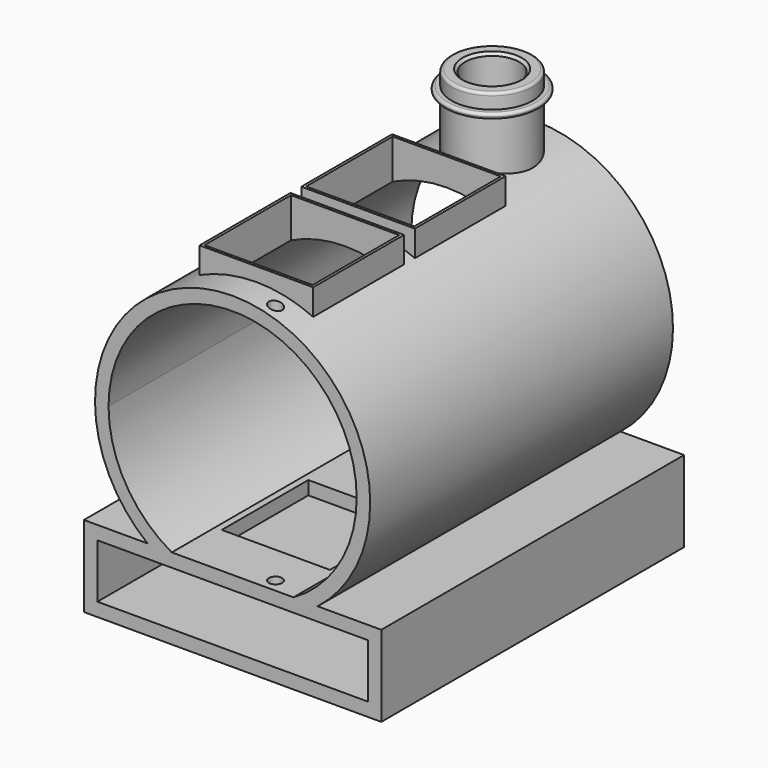
from build123d import *

# Parameters (mm, degrees)
F0_W      = 5
F0_H      = 5
F1_DEPTH  = 140
F5_R      = 15
F5_R_2    = 10
F6_DEPTH  = 30
F7_R      = 10
F8_DEPTH  = 25
F7_W      = 42
F7_H      = 42
F7_W_2    = 40
F7_H_2    = 40
F9_DEPTH  = 10
F10_DEPTH = 25
F11_W     = 40
F11_H     = 40
F11_R     = 2.4384
F11_R_2   = 2.4765
F12_DEPTH = 25
F13_DEPTH = 100
F15_R     = 17.5
F15_R_2   = 10
F16_DEPTH = 2
F17_R     = 0.99999
F18_SIZE  = 1


# Not quite as in the source:
# - a fillet or chamfer is up to 0.001 mm smaller than in the source, because OpenCascade refuses the exact size


with BuildPart() as f1:
    # F0 (on Front) → F1 (new body)
    with BuildSketch(Plane.XZ):
        with BuildLine():
            ThreePointArc((-22.5, -40), (-39.6160493738, -23.1693468188), (-45.8938993767, 0))
            Line((-45.8938993767, 0), (-50.8938993767, 0))
            ThreePointArc((-50.8938993767, 0), (-45.7803505669, -22.233949171), (-31.4672686099, -40))
            Line((-31.4672686099, -40), (-22.5, -40))
        make_face()
        with BuildLine():
            ThreePointArc((-9.0138781887, -45), (-15.954031767, -43.0316031583), (-22.5, -40))
            Line((-22.5, -40), (-31.4672686099, -40))
            ThreePointArc((-31.4672686099, -40), (-27.7333960958, -42.6737358894), (-23.7737038294, -45))
            Line((-23.7737038294, -45), (-9.0138781887, -45))
        make_face()
        with BuildLine():
            ThreePointArc((-45.8938993767, 0), (0, 45.8938993767), (45.8938993767, 0))
            Line((45.8938993767, 0), (50.8938993767, 0))
            ThreePointArc((50.8938993767, 0), (0, 50.8938993767), (-50.8938993767, 0))
            Line((-50.8938993767, 0), (-45.8938993767, 0))
        make_face()
        with BuildLine():
            Line((50.8938993767, 0), (45.8938993767, 0))
            ThreePointArc((45.8938993767, 0), (39.6160493738, -23.1693468188), (22.5, -40))
            Line((22.5, -40), (31.4672686099, -40))
            ThreePointArc((31.4672686099, -40), (45.7803505669, -22.233949171), (50.8938993767, 0))
        make_face()
        with Locations((-52.5, -67.5)):
            Rectangle(F0_W, F0_H)
        with BuildLine():
            ThreePointArc((-23.7737038294, -45), (-27.7333960958, -42.6737358894), (-31.4672686099, -40))
            Line((-31.4672686099, -40), (-55, -40))
            Line((-55, -40), (-55, -65))
            Line((-55, -65), (-50, -65))
            Line((-50, -65), (-50, -45))
            Line((-50, -45), (-23.7737038294, -45))
        make_face()
        with BuildLine():
            Line((55, -40), (31.4672686099, -40))
            ThreePointArc((31.4672686099, -40), (27.7333960958, -42.6737358894), (23.7737038294, -45))
            Line((23.7737038294, -45), (50, -45))
            Line((50, -45), (50, -65))
            Line((50, -65), (-50, -65))
            Line((-50, -65), (-50, -70))
            Line((-50, -70), (55, -70))
            Line((55, -70), (55, -40))
        make_face()
        with BuildLine():
            ThreePointArc((9.0138781887, -45), (15.954031767, -43.0316031583), (22.5, -40))
            Line((22.5, -40), (0, -40))
            Line((0, -40), (-22.5, -40))
            ThreePointArc((-22.5, -40), (-15.954031767, -43.0316031583), (-9.0138781887, -45))
            Line((-9.0138781887, -45), (9.0138781887, -45))
        make_face()
        with BuildLine():
            Line((31.4672686099, -40), (22.5, -40))
            ThreePointArc((22.5, -40), (15.954031767, -43.0316031583), (9.0138781887, -45))
            Line((9.0138781887, -45), (23.7737038294, -45))
            ThreePointArc((23.7737038294, -45), (27.7333960958, -42.6737358894), (31.4672686099, -40))
        make_face()
    extrude(amount=F1_DEPTH)

    # F5 (on offset) → F6 (join)
    with BuildSketch(Plane.XY.offset(76)):
        with Locations((0, -20)):
            Circle(F5_R)
        with Locations((0, -20)):
            Circle(F5_R_2, mode=Mode.SUBTRACT)
    extrude(amount=-F6_DEPTH)

    # F7 (on offset) → F8 (cut)
    with BuildSketch(Plane.XY.offset(56)):
        with Locations((0, -20)):
            Circle(F7_R)
    extrude(amount=-F8_DEPTH, mode=Mode.SUBTRACT)

    # F7 (on offset) → F9 (join)
    with BuildSketch(Plane.XY.offset(56)):
        with Locations((0, -61)):
            Rectangle(F7_W, F7_H)
        with Locations((0, -61)):
            Rectangle(F7_W_2, F7_H_2, mode=Mode.SUBTRACT)
        with Locations((0, -108)):
            Rectangle(F7_W, F7_H)
        with Locations((0, -108)):
            Rectangle(F7_W_2, F7_H_2, mode=Mode.SUBTRACT)
    extrude(amount=-F9_DEPTH)

    # F7 (on offset) → F10 (cut)
    with BuildSketch(Plane.XY.offset(56)):
        with Locations((0, -61)):
            Rectangle(F7_W_2, F7_H_2)
        with Locations((0, -108)):
            Rectangle(F7_W_2, F7_H_2)
    extrude(amount=-F10_DEPTH, mode=Mode.SUBTRACT)

    # F11 (on face) → F12 (cut)
    with BuildSketch(Plane(origin=(0, 0, -45), x_dir=(1, 0, 0), z_dir=(0, 0, -1))):
        with Locations((3.8294e-06, 40)):
            Rectangle(F11_W, F11_H)
        with Locations((0, 100)):
            Rectangle(F11_W, F11_H)
        with Locations((0, 70)):
            Circle(F11_R)
        with Locations((11.8868519147, 135)):
            Circle(F11_R_2)
    extrude(amount=-F12_DEPTH, mode=Mode.SUBTRACT)

    # F11 (on face) → F13 (cut)
    with BuildSketch(Plane(origin=(0, 0, -45), x_dir=(1, 0, 0), z_dir=(0, 0, -1))):
        with Locations((11.8868519147, 135)):
            Circle(F11_R_2)
    extrude(amount=-F13_DEPTH, mode=Mode.SUBTRACT)

    # F15 (on offset) → F16 (join)
    with BuildSketch(Plane.XY.offset(68.5)):
        with Locations((0, -20)):
            Circle(F15_R)
        with Locations((0, -20)):
            Circle(F15_R_2, mode=Mode.SUBTRACT)
    extrude(amount=F16_DEPTH)

    # F17 (radius 1 in the source; OpenCascade refuses exactly that, so slightly less here)
    f17_edges = [f1.edges().sort_by_distance(p)[0] for p in [
        (-17.5, -20, 70.5),
        (-17.5, -20, 68.5),
        (-15, -20, 76),
    ]]
    fillet(f17_edges, radius=F17_R)

    # F18
    f18_edges = [f1.edges().sort_by_distance(p)[0] for p in [
        (-10, -20, 76),
    ]]
    chamfer(f18_edges, length=F18_SIZE)


solid = f1.part
